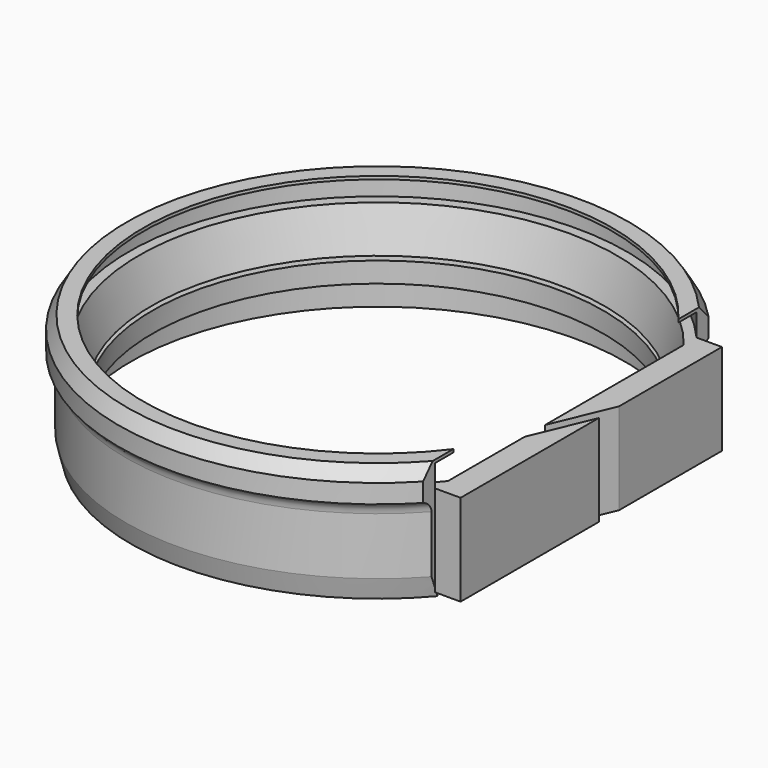
from build123d import *

# Parameters (mm, degrees)
F0_W      = 1.4
F0_H      = 0.3
F0_W_2    = 2
F0_H_2    = 2
F4_SIZE2  = 0.49999
F4_SIZE   = 1.99999
F5_R      = 0.5
F7_DEPTH  = 25
F9_DEPTH  = 9
F11_DEPTH = 100


# Not quite as in the source:
# - a fillet or chamfer that OpenCascade refuses, or shapes differently, is made with other operations: its cross-section is extruded or revolved along the edge and cut away or added
# - a fillet or chamfer is up to 0.001 mm smaller than in the source, because OpenCascade refuses the exact size


with BuildPart() as f1:
    # F0 (on Front) → F1 (revolve)
    with BuildSketch(Plane.XZ):
        Polygon((-24.5, 0), (-25.5, 0), (-25.5, -3.1555826106), (-24.8, -3.1555826106), (-24.8, -11.9555826106), (-24.3, -11.9555826106), (-24.3, -4.9555826106), (-23.391673381, -4.9555826106), (-22.9283481642, -6.5), (-22.3, -6.5), (-23.5, -2.5), (-24.5, -2.5), (-24.5, -0.3), align=None)
        with Locations((-23.8, -0.15)):
            Rectangle(F0_W, F0_H)
    revolve(axis=Axis((0, 0, 1.0689813644), (0, 0, -1)))

    # F2: chamfer of 0.8 x 1.3 on 1 edges, made by hand

    # F2_s1 → F2_t2 (revolve, cut)
    with BuildSketch(Plane.XZ):
        Polygon((-25.5, -1.3), (-24.7, 0), (-25.5, 0), align=None)
    revolve(axis=Axis((0, 0, 0), (0, 0, -1)), mode=Mode.SUBTRACT)

    # F3: fillet of radius 1.4 on 1 edges, made by hand

    # F3_s1 → F3_t2 (revolve)
    with BuildSketch(Plane.XZ):
        with BuildLine():
            ThreePointArc((-25.4997998621, -3.1552362801), (-24.9872079854, -3.6681342757), (-24.7996, -4.3685755865))
            Line((-24.7996, -4.3685755865), (-24.6594634315, -4.3685755865))
            ThreePointArc((-24.6594634315, -4.3685755865), (-24.6598634315, -3.7620790985), (-24.6598634315, -3.1555826106))
            Line((-24.6598634315, -3.1555826106), (-24.8, -3.015446042))
            ThreePointArc((-24.8, -3.015446042), (-25.1498999311, -3.015446042), (-25.4296832798, -3.0339023494))
            Line((-25.4296832798, -3.0339023494), (-25.4997998621, -3.1552362801))
        make_face()
    revolve(axis=Axis((0, 0, -3.1555826106), (0, 0, -1)))

    # F4 (size 2 and 0.5 in the source; OpenCascade refuses exactly that, so slightly less here)
    f4_edges = [f1.edges().sort_by_distance(p)[0] for p in [
        (24.8, 0, -11.955583),
    ]]
    chamfer(f4_edges, length=F4_SIZE, length2=F4_SIZE2)

    # F5
    f5_edges = [f1.edges().sort_by_distance(p)[0] for p in [
        (23.391673, 0, -4.955583),
    ]]
    fillet(f5_edges, radius=F5_R)


with BuildPart() as f1b:
    # F0 (on Front) → F1, piece 2 (revolve)
    with BuildSketch(Plane.XZ):
        with Locations((-23.2, -7.8631715626)):
            Rectangle(F0_W_2, F0_H_2)
    revolve(axis=Axis((0, 0, 1.0689813644), (0, 0, -1)))


with BuildPart() as f7_tool:
    # F6 (on Top) → F7 (new body)
    with BuildSketch(Plane.XY):
        Polygon((18.4932420089, 17.5570498661), (18.4932420089, 14.5), (18.4932420089, -14.5), (18.4932420089, -17.5570498661), (23.4932420089, -17.5570498661), (23.4932420089, 17.5570498661), align=None)
        Polygon((18.4932420089, 29.2936375588), (18.4932420089, 17.5570498661), (23.4932420089, 17.5570498661), (23.4932420089, -17.5570498661), (18.4932420089, -17.5570498661), (18.4932420089, -27.3348336816), (60.3667099652, -27.3348336816), (60.3667099652, 29.2936375588), align=None)
    extrude(amount=-F7_DEPTH)


with BuildPart() as f1_1:
    add(f1.part)

    # F7: cut by f7_tool
    add(f7_tool.part, mode=Mode.SUBTRACT)



with BuildPart() as f1b_1:
    add(f1b.part)

    # F7: cut by f7_tool
    add(f7_tool.part, mode=Mode.SUBTRACT)


with BuildPart() as f1_2:
    add(f1_1.part)

    add(f1b_1.part)  # F9 merges F1b
    # F8 (on face) → F9 (join)
    with BuildSketch(Plane.XY.offset(-2.5)):
        Polygon((20.9932420089, 16.07015868), (18.4932420089, 16.07015868), (18.4932420089, 14.5), (18.4932420089, -14.5), (18.4932420089, -16.07015868), (20.9932420089, -16.07015868), align=None)
    extrude(amount=-F9_DEPTH)

    # F10 (on Top) → F11 (cut)
    with BuildSketch(Plane.XY):
        Polygon((28.4932420089, 21.42984132), (15.9932420089, -8.57015868), (15.9932420089, -11.07015868), (28.4932420089, 18.92984132), align=None)
    extrude(amount=-F11_DEPTH, mode=Mode.SUBTRACT)


solid = f1_2.part
